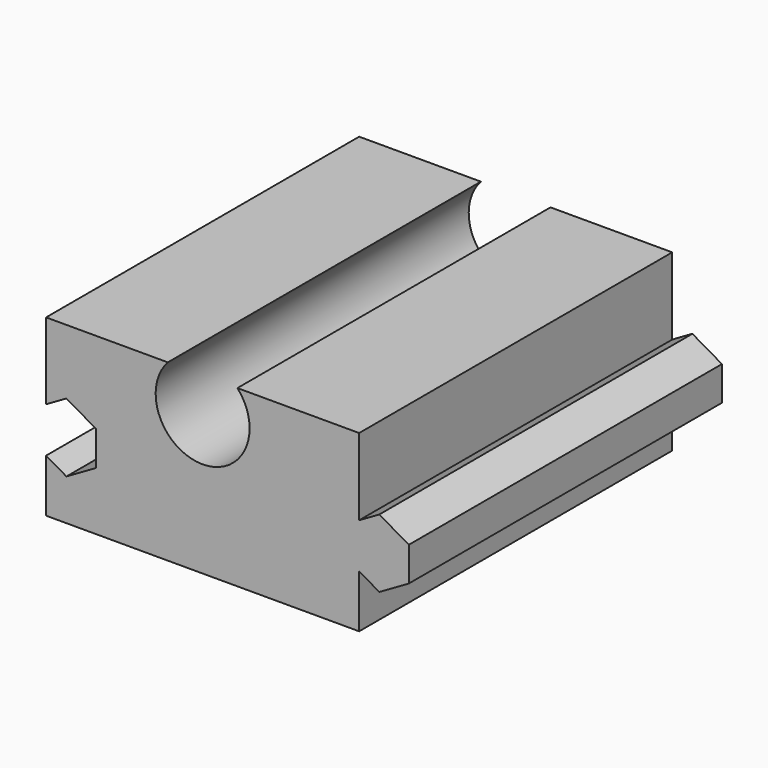
from build123d import *

# Parameters (mm, degrees)
F1_DEPTH = 25


# Not quite as in the source:
# - a feature names something its author has since deleted; it is built from what else it names


with BuildPart() as f1:
    # F0 (on Front) → F1 (new body)
    with BuildSketch(Plane.XZ):
        with BuildLine():
            Line((-10, -5.576437097), (10, -5.576437097))
            Line((10, -5.576437097), (10, -2.201012618))
            Line((10, -2.201012618), (9.4, -1.8546024565))
            Line((9.4, -1.8546024565), (9.4, 0.3245011641))
            Line((9.4, 0.3245011641), (10, 0.6709113256))
            Line((10, 0.6709113256), (10, 5.576437097))
            Line((10, 5.576437097), (2.2236531144, 5.576437097))
            ThreePointArc((2.2236531144, 5.576437097), (2.7991926821, 4.6417723907), (3, 3.5626429599))
            ThreePointArc((3, 3.5626429599), (-1.0791294308, 0.7634502778), (-2.2236531144, 5.576437097))
            Line((-2.2236531144, 5.576437097), (-10, 5.576437097))
            Line((-10, 5.576437097), (-10, 0.6884473353))
            Line((-10, 0.6884473353), (-8.6999533325, 1.4390296287))
            Line((-8.6999533325, 1.4390296287), (-6.7999051139, 0.3420362782))
            Line((-6.7999051139, 0.3420362782), (-6.7999051139, -1.8519504229))
            Line((-6.7999051139, -1.8519504229), (-8.6999533325, -2.9489437734))
            Line((-8.6999533325, -2.9489437734), (-10, -2.19836148))
            Line((-10, -2.19836148), (-10, -5.576437097))
        make_face()
        Polygon((10, 0.6709113256), (10, -2.201012618), (11.2871590928, -2.9441542667), (13.1743181857, -1.8546024565), (13.1743181857, 0.3245011641), (11.2871590928, 1.4140529743), align=None)
        Polygon((9.4, -1.8546024565), (10, -2.201012618), (10, 0.6709113256), (9.4, 0.3245011641), align=None)
    extrude(amount=F1_DEPTH)


solid = f1.part
